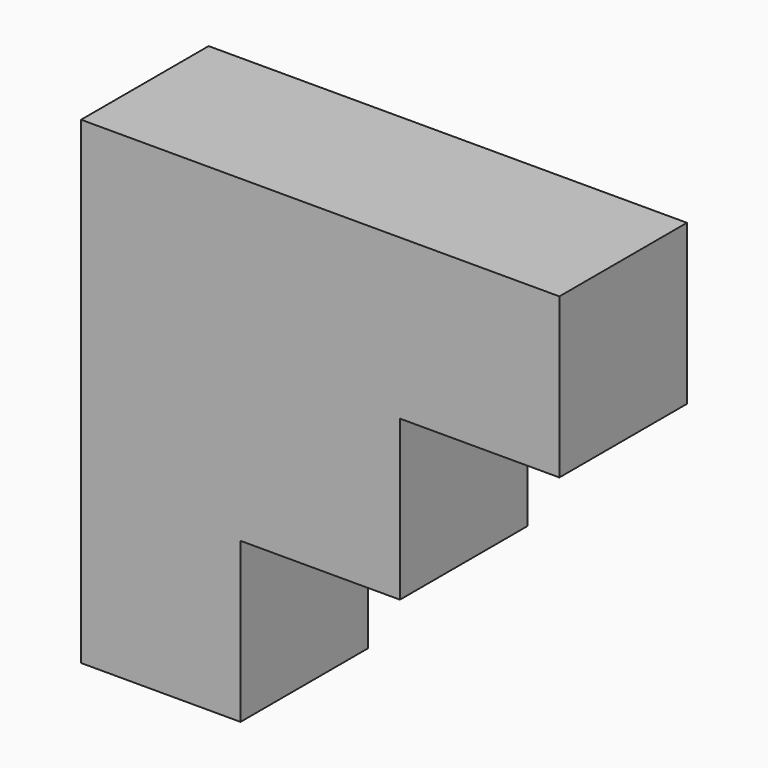
from build123d import *

# Parameters (mm, degrees)
F1_W     = 228.6
F1_H     = 228.6
F2_DEPTH = 76.2
F3_W     = 76.2
F3_H     = 76.2
F4_DEPTH = 76.201


# Not quite as in the source:
# - a variable given as a bare number and used for a length is read in inches; the dataset says mm whatever the document's units were


with BuildPart() as f2:
    # F1 (on Front) → F2 (new body)
    with BuildSketch(Plane.XZ):
        Rectangle(F1_W, F1_H)
    extrude(amount=F2_DEPTH)

    # F3 (on face) → F4 (cut, through all)
    with BuildSketch(Plane.XZ.offset(76.2)):
        with Locations((76.2, -76.2)):
            Rectangle(F3_W, F3_H)
        with Locations((0, -76.2)):
            Rectangle(F3_W, F3_H)
        with Locations((76.2, 0)):
            Rectangle(F3_W, F3_H)
    extrude(amount=-F4_DEPTH, mode=Mode.SUBTRACT)


solid = f2.part
